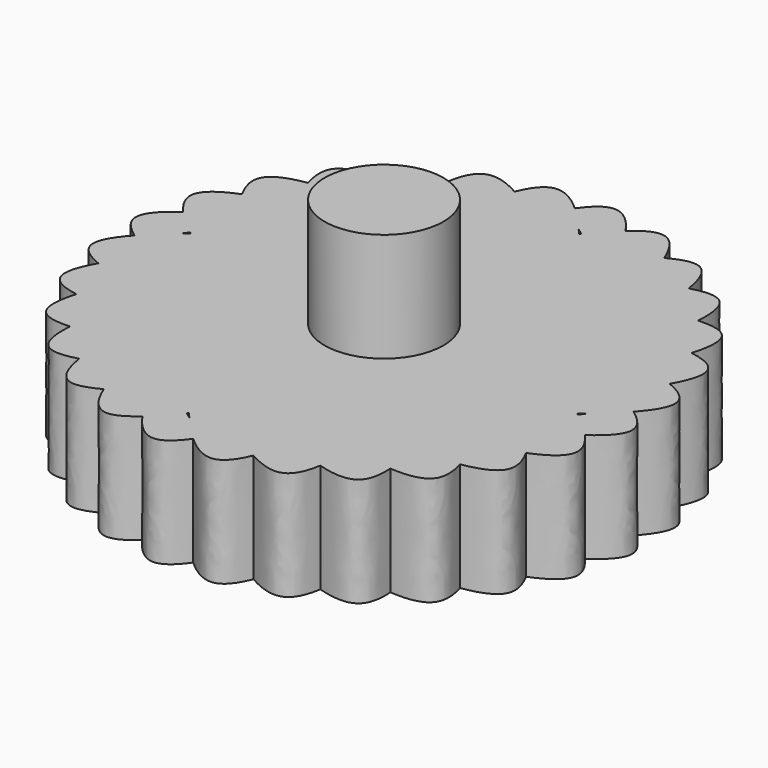
from build123d import *

# Parameters (mm, degrees)
F1_DEPTH = 25.4
F2_COUNT = 7
F3_R     = 5.08
F5_DEPTH = 25.4
F6_R     = 13.8422329742
F7_DEPTH = 25.4
F8_COUNT = 4


with BuildPart() as f1:
    # F0 (on Top) → F1 (new body)
    with BuildSketch(Plane.XY):
        with BuildLine():
            ThreePointArc((-0.3036099023, 41.7036828128), (-29.3821999901, -29.5968860332), (41.704787964, 0))
            ThreePointArc((41.704787964, 0), (38.5508515564, 15.909782632), (29.5660770028, 29.4132016242))
            ThreePointArc((29.5660770028, 29.4132016242), (15.869372299, 38.5675039633), (-0.3036099023, 41.7036828128))
        make_face()
        with BuildLine():
            ThreePointArc((-0.3036099023, 41.7036828128), (15.869372299, 38.5675039633), (29.5660770028, 29.4132016242))
            add(Edge.make_bspline(
                [(-0.3036099023, 41.7036828128), (6.4916545945, 50.8782567936), (20.9015792408, 70.3101588182), (26.5683495721, 43.5511495821), (29.5660770028, 29.4132016242)],
                knots=[0, 0, 0, 0, 0.4717280628, 1, 1, 1, 1], degree=3))
        make_face()
    extrude(amount=F1_DEPTH)

    # F2: F1 ×7 about axis
    f2_axis = Axis((0, 0, 25.4), (0, 0, -1))


with BuildPart() as f1_1:
    add(f1.part)
    for i in range(1, F2_COUNT):
        add(f1.part.rotate(f2_axis, i * 360 / F2_COUNT))

    # F3
    f3_edges = [f1_1.edges().sort_by_distance(p)[0] for p in [
        (-0.30361, 41.703683, 12.7),
    ]]
    fillet(f3_edges, radius=F3_R)

    # F4 (on face) → F5 (cut)
    with BuildSketch(Plane.XY.offset(25.4)):
        with BuildLine():
            add(Edge.make_bspline(
                [(-36.3872498274, -6.7111928947), (-41.8735206701, -9.5542377544), (-62.7340181989, 2.2079607061), (-29.4439624143, 18.5836450682), (-31.0447006553, -3.9426261585), (-36.3872498274, -6.7111928947)],
                knots=[0, 0, 0, 0, 0.3333906433, 0.6753430597, 1, 1, 1, 1], degree=3))
        make_face()
    extrude(amount=-F5_DEPTH, mode=Mode.SUBTRACT)

    # F6 (on face) → F7 (join)
    with BuildSketch(Plane.XY.offset(25.4)):
        Circle(F6_R)
    extrude(amount=F7_DEPTH)

    # F8: F1 ×4 about axis
    f8_axis = Axis((0, 0, 50.8), (0, 0, 1))


with BuildPart() as f1_2:
    add(f1_1.part)
    for i in range(1, F8_COUNT):
        add(f1_1.part.rotate(f8_axis, i * 360 / F8_COUNT))


solid = f1_2.part
